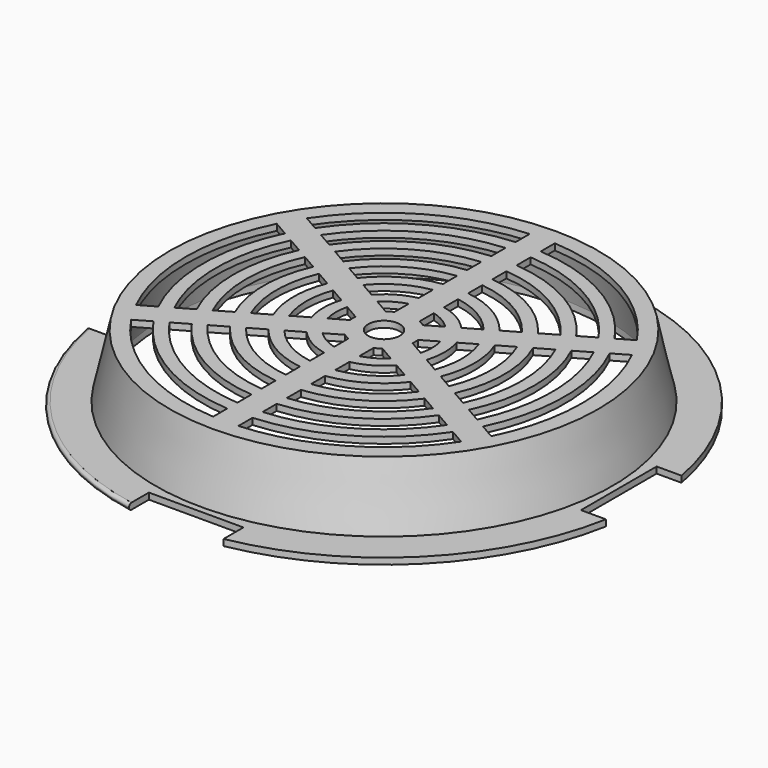
from build123d import *

# Parameters (mm, degrees)
F2_T      = -2.54
F3_R      = 106.3625
F3_R_2    = 89.4715
F4_DEPTH  = 2.54
F6_DEPTH  = 27.941
F7_W      = 25.2537746336
F7_H      = 38.1
F7_W_2    = 38.1
F7_H_2    = 25.2537746336
F8_DEPTH  = 27.941
F9_R      = 6.35
F10_DEPTH = 27.941
F11_R     = 1.26999


# Not quite as in the source:
# - a fillet or chamfer is up to 0.001 mm smaller than in the source, because OpenCascade refuses the exact size


with BuildPart() as f1:
    # F0 (on Front) → F1 (revolve)
    with BuildSketch(Plane.XZ):
        Polygon((-92.075, 0), (0, 0), (0, 25.4), (-86.36, 25.4), align=None)
    revolve(axis=Axis((0, 0, 34.7240492702), (0, 0, 1)))

    # F2
    f2_openings = [f1.faces().sort_by_distance(p)[0] for p in [
        (0, 0, 0),
    ]]
    offset(amount=F2_T, openings=f2_openings)

    # F3 (on face) → F4 (join)
    with BuildSketch(Plane(origin=(0, 0, 0), x_dir=(1, 0, 0), z_dir=(0, 0, -1))):
        Circle(F3_R)
        Circle(F3_R_2, mode=Mode.SUBTRACT)
    extrude(amount=F4_DEPTH)

    # F5 (on face) → F6 (cut, through all)
    with BuildSketch(Plane.XY.offset(25.4)):
        with BuildLine():
            Line((5.08, 30.9437422652), (5.08, 23.8317422652))
            ThreePointArc((5.08, 23.8317422652), (12.1835784911, 21.1025769646), (18.0988942181, 16.3152801838))
            Line((18.0988942181, 16.3152801838), (24.2580668898, 19.8712801838))
            ThreePointArc((24.2580668898, 19.8712801838), (15.678979442, 27.1567890044), (5.08, 30.9437422652))
        make_face()
        with BuildLine():
            ThreePointArc((13.6994851669, 13.7752801838), (9.7138334089, 16.8248530004), (5.08, 18.7517422652))
            Line((5.08, 18.7517422652), (5.08, 11.6397422652))
            ThreePointArc((5.08, 11.6397422652), (6.35, 10.9985226281), (7.5403124952, 10.2192801838))
            Line((7.5403124952, 10.2192801838), (13.6994851669, 13.7752801838))
        make_face()
        with BuildLine():
            Line((5.08, 43.1357422652), (5.08, 36.0237422652))
            ThreePointArc((5.08, 36.0237422652), (18.1900825094, 31.5061471001), (28.657475941, 22.4112801838))
            Line((28.657475941, 22.4112801838), (34.8166486128, 25.9672801838))
            ThreePointArc((34.8166486128, 25.9672801838), (21.716921172, 37.6148108539), (5.08, 43.1357422652))
        make_face()
        with BuildLine():
            Line((5.08, 55.3277422652), (5.08, 48.2157422652))
            ThreePointArc((5.08, 48.2157422652), (24.2413087631, 41.9871784196), (39.216057664, 28.5072801838))
            Line((39.216057664, 28.5072801838), (45.3752303357, 32.0632801838))
            ThreePointArc((45.3752303357, 32.0632801838), (27.7802333691, 48.1167756414), (5.08, 55.3277422652))
        make_face()
        with BuildLine():
            ThreePointArc((-5.08, 55.3277422652), (-27.7802333691, 48.1167756414), (-45.3752303357, 32.0632801838))
            Line((-45.3752303357, 32.0632801838), (-39.216057664, 28.5072801838))
            ThreePointArc((-39.216057664, 28.5072801838), (-24.2413087631, 41.9871784196), (-5.08, 48.2157422652))
            Line((-5.08, 48.2157422652), (-5.08, 55.3277422652))
        make_face()
        with BuildLine():
            Line((-34.8166486128, 25.9672801838), (-28.657475941, 22.4112801838))
            ThreePointArc((-28.657475941, 22.4112801838), (-18.1900825094, 31.5061471001), (-5.08, 36.0237422652))
            Line((-5.08, 36.0237422652), (-5.08, 43.1357422652))
            ThreePointArc((-5.08, 43.1357422652), (-21.716921172, 37.6148108539), (-34.8166486128, 25.9672801838))
        make_face()
        with BuildLine():
            ThreePointArc((-5.08, 30.9437422652), (-15.678979442, 27.1567890044), (-24.2580668898, 19.8712801838))
            Line((-24.2580668898, 19.8712801838), (-18.0988942181, 16.3152801838))
            ThreePointArc((-18.0988942181, 16.3152801838), (-12.1835784911, 21.1025769646), (-5.08, 23.8317422652))
            Line((-5.08, 23.8317422652), (-5.08, 30.9437422652))
        make_face()
        with BuildLine():
            ThreePointArc((-5.08, 18.7517422652), (-9.7138334089, 16.8248530004), (-13.6994851669, 13.7752801838))
            Line((-13.6994851669, 13.7752801838), (-7.5403124952, 10.2192801838))
            ThreePointArc((-7.5403124952, 10.2192801838), (-6.35, 10.9985226281), (-5.08, 11.6397422652))
            Line((-5.08, 11.6397422652), (-5.08, 18.7517422652))
        make_face()
        with BuildLine():
            ThreePointArc((-50.4552303357, 23.2644620814), (-55.5604667382, 0), (-50.4552303357, -23.2644620814))
            Line((-50.4552303357, -23.2644620814), (-44.296057664, -19.7084620814))
            ThreePointArc((-44.296057664, -19.7084620814), (-48.4826175261, 0), (-44.296057664, 19.7084620814))
            Line((-44.296057664, 19.7084620814), (-50.4552303357, 23.2644620814))
        make_face()
        with BuildLine():
            Line((-39.8966486128, -17.1684620814), (-33.737475941, -13.6124620814))
            ThreePointArc((-33.737475941, -13.6124620814), (-36.3801650187, 0), (-33.737475941, 13.6124620814))
            Line((-33.737475941, 13.6124620814), (-39.8966486128, 17.1684620814))
            ThreePointArc((-39.8966486128, 17.1684620814), (-43.4338423441, 0), (-39.8966486128, -17.1684620814))
        make_face()
        with BuildLine():
            ThreePointArc((-29.3380668898, 11.0724620814), (-31.3579588841, 0), (-29.3380668898, -11.0724620814))
            Line((-29.3380668898, -11.0724620814), (-23.1788942181, -7.5164620814))
            ThreePointArc((-23.1788942181, -7.5164620814), (-24.3671569822, 0), (-23.1788942181, 7.5164620814))
            Line((-23.1788942181, 7.5164620814), (-29.3380668898, 11.0724620814))
        make_face()
        with BuildLine():
            ThreePointArc((-18.7794851669, 4.9764620814), (-19.4276668177, 0), (-18.7794851669, -4.9764620814))
            Line((-18.7794851669, -4.9764620814), (-12.6203124952, -1.4204620814))
            ThreePointArc((-12.6203124952, -1.4204620814), (-12.7, 0), (-12.6203124952, 1.4204620814))
            Line((-12.6203124952, 1.4204620814), (-18.7794851669, 4.9764620814))
        make_face()
        with BuildLine():
            ThreePointArc((-45.3752303357, -32.0632801838), (-27.7802333691, -48.1167756414), (-5.08, -55.3277422652))
            Line((-5.08, -55.3277422652), (-5.08, -48.2157422652))
            ThreePointArc((-5.08, -48.2157422652), (-24.2413087631, -41.9871784196), (-39.216057664, -28.5072801838))
            Line((-39.216057664, -28.5072801838), (-45.3752303357, -32.0632801838))
        make_face()
        with BuildLine():
            Line((-5.08, -43.1357422652), (-5.08, -36.0237422652))
            ThreePointArc((-5.08, -36.0237422652), (-18.1900825094, -31.5061471001), (-28.657475941, -22.4112801838))
            Line((-28.657475941, -22.4112801838), (-34.8166486128, -25.9672801838))
            ThreePointArc((-34.8166486128, -25.9672801838), (-21.716921172, -37.6148108539), (-5.08, -43.1357422652))
        make_face()
        with BuildLine():
            ThreePointArc((-24.2580668898, -19.8712801838), (-15.678979442, -27.1567890044), (-5.08, -30.9437422652))
            Line((-5.08, -30.9437422652), (-5.08, -23.8317422652))
            ThreePointArc((-5.08, -23.8317422652), (-12.1835784911, -21.1025769646), (-18.0988942181, -16.3152801838))
            Line((-18.0988942181, -16.3152801838), (-24.2580668898, -19.8712801838))
        make_face()
        with BuildLine():
            ThreePointArc((-13.6994851669, -13.7752801838), (-9.7138334089, -16.8248530004), (-5.08, -18.7517422652))
            Line((-5.08, -18.7517422652), (-5.08, -11.6397422652))
            ThreePointArc((-5.08, -11.6397422652), (-6.35, -10.9985226281), (-7.5403124952, -10.2192801838))
            Line((-7.5403124952, -10.2192801838), (-13.6994851669, -13.7752801838))
        make_face()
        with BuildLine():
            ThreePointArc((5.08, -55.3277422652), (27.7802333691, -48.1167756414), (45.3752303357, -32.0632801838))
            Line((45.3752303357, -32.0632801838), (39.216057664, -28.5072801838))
            ThreePointArc((39.216057664, -28.5072801838), (24.2413087631, -41.9871784196), (5.08, -48.2157422652))
            Line((5.08, -48.2157422652), (5.08, -55.3277422652))
        make_face()
        with BuildLine():
            Line((34.8166486128, -25.9672801838), (28.657475941, -22.4112801838))
            ThreePointArc((28.657475941, -22.4112801838), (18.1900825094, -31.5061471001), (5.08, -36.0237422652))
            Line((5.08, -36.0237422652), (5.08, -43.1357422652))
            ThreePointArc((5.08, -43.1357422652), (21.716921172, -37.6148108539), (34.8166486128, -25.9672801838))
        make_face()
        with BuildLine():
            ThreePointArc((5.08, -30.9437422652), (15.678979442, -27.1567890044), (24.2580668898, -19.8712801838))
            Line((24.2580668898, -19.8712801838), (18.0988942181, -16.3152801838))
            ThreePointArc((18.0988942181, -16.3152801838), (12.1835784911, -21.1025769646), (5.08, -23.8317422652))
            Line((5.08, -23.8317422652), (5.08, -30.9437422652))
        make_face()
        with BuildLine():
            ThreePointArc((5.08, -18.7517422652), (9.7138334089, -16.8248530004), (13.6994851669, -13.7752801838))
            Line((13.6994851669, -13.7752801838), (7.5403124952, -10.2192801838))
            ThreePointArc((7.5403124952, -10.2192801838), (6.35, -10.9985226281), (5.08, -11.6397422652))
            Line((5.08, -11.6397422652), (5.08, -18.7517422652))
        make_face()
        with BuildLine():
            ThreePointArc((50.4552303357, -23.2644620814), (55.5604667382, 0), (50.4552303357, 23.2644620814))
            Line((50.4552303357, 23.2644620814), (44.296057664, 19.7084620814))
            ThreePointArc((44.296057664, 19.7084620814), (48.4826175261, 0), (44.296057664, -19.7084620814))
            Line((44.296057664, -19.7084620814), (50.4552303357, -23.2644620814))
        make_face()
        with BuildLine():
            Line((39.8966486128, 17.1684620814), (33.737475941, 13.6124620814))
            ThreePointArc((33.737475941, 13.6124620814), (36.3801650187, 0), (33.737475941, -13.6124620814))
            Line((33.737475941, -13.6124620814), (39.8966486128, -17.1684620814))
            ThreePointArc((39.8966486128, -17.1684620814), (43.4338423441, 0), (39.8966486128, 17.1684620814))
        make_face()
        with BuildLine():
            ThreePointArc((29.3380668898, -11.0724620814), (31.3579588841, 0), (29.3380668898, 11.0724620814))
            Line((29.3380668898, 11.0724620814), (23.1788942181, 7.5164620814))
            ThreePointArc((23.1788942181, 7.5164620814), (24.3671569822, 0), (23.1788942181, -7.5164620814))
            Line((23.1788942181, -7.5164620814), (29.3380668898, -11.0724620814))
        make_face()
        with BuildLine():
            ThreePointArc((18.7794851669, -4.9764620814), (19.4276668177, 0), (18.7794851669, 4.9764620814))
            Line((18.7794851669, 4.9764620814), (12.6203124952, 1.4204620814))
            ThreePointArc((12.6203124952, 1.4204620814), (12.7, 0), (12.6203124952, -1.4204620814))
            Line((12.6203124952, -1.4204620814), (18.7794851669, -4.9764620814))
        make_face()
        with BuildLine():
            Line((5.08, 67.5197422652), (5.08, 60.4077422652))
            ThreePointArc((5.08, 60.4077422652), (30.3104838529, 52.4992980351), (49.7746393869, 34.6032801838))
            Line((49.7746393869, 34.6032801838), (55.9338120586, 38.1592801838))
            ThreePointArc((55.9338120586, 38.1592801838), (33.8552876061, 58.6390782386), (5.08, 67.5197422652))
        make_face()
        with BuildLine():
            Line((5.08, 79.7117422652), (5.08, 72.5997422652))
            ThreePointArc((5.08, 72.5997422652), (36.3886279522, 63.0269524309), (60.3332211099, 40.6992801838))
            Line((60.3332211099, 40.6992801838), (66.4923937816, 44.2552801838))
            ThreePointArc((66.4923937816, 44.2552801838), (39.9367257513, 69.1724380893), (5.08, 79.7117422652))
        make_face()
        with BuildLine():
            Line((-55.9338120586, 38.1592801838), (-49.7746393869, 34.6032801838))
            ThreePointArc((-49.7746393869, 34.6032801838), (-30.3104838529, 52.4992980351), (-5.08, 60.4077422652))
            Line((-5.08, 60.4077422652), (-5.08, 67.5197422652))
            ThreePointArc((-5.08, 67.5197422652), (-33.8552876061, 58.6390782386), (-55.9338120586, 38.1592801838))
        make_face()
        with BuildLine():
            ThreePointArc((-60.3332211099, 40.6992801838), (-36.3886279522, 63.0269524309), (-5.08, 72.5997422652))
            Line((-5.08, 72.5997422652), (-5.08, 79.7117422652))
            ThreePointArc((-5.08, 79.7117422652), (-39.9367257513, 69.1724380893), (-66.4923937816, 44.2552801838))
            Line((-66.4923937816, 44.2552801838), (-60.3332211099, 40.6992801838))
        make_face()
        with BuildLine():
            Line((-61.0138120586, -29.3604620814), (-54.8546393869, -25.8044620814))
            ThreePointArc((-54.8546393869, -25.8044620814), (-60.6209677057, 0), (-54.8546393869, 25.8044620814))
            Line((-54.8546393869, 25.8044620814), (-61.0138120586, 29.3604620814))
            ThreePointArc((-61.0138120586, 29.3604620814), (-67.7105752121, 0), (-61.0138120586, -29.3604620814))
        make_face()
        with BuildLine():
            ThreePointArc((-65.4132211099, -31.9004620814), (-72.7772559044, 0), (-65.4132211099, 31.9004620814))
            Line((-65.4132211099, 31.9004620814), (-71.5723937816, 35.4564620814))
            ThreePointArc((-71.5723937816, 35.4564620814), (-79.8734515027, 0), (-71.5723937816, -35.4564620814))
            Line((-71.5723937816, -35.4564620814), (-65.4132211099, -31.9004620814))
        make_face()
        with BuildLine():
            Line((-5.08, -67.5197422652), (-5.08, -60.4077422652))
            ThreePointArc((-5.08, -60.4077422652), (-30.3104838529, -52.4992980351), (-49.7746393869, -34.6032801838))
            Line((-49.7746393869, -34.6032801838), (-55.9338120586, -38.1592801838))
            ThreePointArc((-55.9338120586, -38.1592801838), (-33.8552876061, -58.6390782386), (-5.08, -67.5197422652))
        make_face()
        with BuildLine():
            ThreePointArc((-5.08, -72.5997422652), (-36.3886279522, -63.0269524309), (-60.3332211099, -40.6992801838))
            Line((-60.3332211099, -40.6992801838), (-66.4923937816, -44.2552801838))
            ThreePointArc((-66.4923937816, -44.2552801838), (-39.9367257513, -69.1724380893), (-5.08, -79.7117422652))
            Line((-5.08, -79.7117422652), (-5.08, -72.5997422652))
        make_face()
        with BuildLine():
            Line((55.9338120586, -38.1592801838), (49.7746393869, -34.6032801838))
            ThreePointArc((49.7746393869, -34.6032801838), (30.3104838529, -52.4992980351), (5.08, -60.4077422652))
            Line((5.08, -60.4077422652), (5.08, -67.5197422652))
            ThreePointArc((5.08, -67.5197422652), (33.8552876061, -58.6390782386), (55.9338120586, -38.1592801838))
        make_face()
        with BuildLine():
            ThreePointArc((60.3332211099, -40.6992801838), (36.3886279522, -63.0269524309), (5.08, -72.5997422652))
            Line((5.08, -72.5997422652), (5.08, -79.7117422652))
            ThreePointArc((5.08, -79.7117422652), (39.9367257513, -69.1724380893), (66.4923937816, -44.2552801838))
            Line((66.4923937816, -44.2552801838), (60.3332211099, -40.6992801838))
        make_face()
        with BuildLine():
            Line((61.0138120586, 29.3604620814), (54.8546393869, 25.8044620814))
            ThreePointArc((54.8546393869, 25.8044620814), (60.6209677057, 0), (54.8546393869, -25.8044620814))
            Line((54.8546393869, -25.8044620814), (61.0138120586, -29.3604620814))
            ThreePointArc((61.0138120586, -29.3604620814), (67.7105752121, 0), (61.0138120586, 29.3604620814))
        make_face()
        with BuildLine():
            ThreePointArc((65.4132211099, 31.9004620814), (72.7772559044, 0), (65.4132211099, -31.9004620814))
            Line((65.4132211099, -31.9004620814), (71.5723937816, -35.4564620814))
            ThreePointArc((71.5723937816, -35.4564620814), (79.8734515027, 0), (71.5723937816, 35.4564620814))
            Line((71.5723937816, 35.4564620814), (65.4132211099, 31.9004620814))
        make_face()
    extrude(amount=-F6_DEPTH, mode=Mode.SUBTRACT)

    # F7 (on face) → F8 (cut, through all)
    with BuildSketch(Plane(origin=(0, 0, -2.54), x_dir=(1, 0, 0), z_dir=(0, 0, -1))):
        with Locations((-107.2418873168, 0)):
            Rectangle(F7_W, F7_H)
        with Locations((107.2418873168, 0)):
            Rectangle(F7_W, F7_H)
        with Locations((0, -107.2418873168)):
            Rectangle(F7_W_2, F7_H_2)
        with Locations((0, 107.2418873168)):
            Rectangle(F7_W_2, F7_H_2)
    extrude(amount=-F8_DEPTH, mode=Mode.SUBTRACT)

    # F9 (on face) → F10 (cut, through all)
    with BuildSketch(Plane.XY.offset(25.4)):
        Circle(F9_R)
    extrude(amount=-F10_DEPTH, mode=Mode.SUBTRACT)

    # F11 (radius 1.27 in the source; OpenCascade refuses exactly that, so slightly less here)
    f11_edges = [f1.edges().sort_by_distance(p)[0] for p in [
        (-75.209645, 75.209645, -2.54),
        (-75.209645, 75.209645, 0),
        (-75.209645, -75.209645, 0),
        (-75.209645, -75.209645, -2.54),
    ]]
    fillet(f11_edges, radius=F11_R)


solid = f1.part
